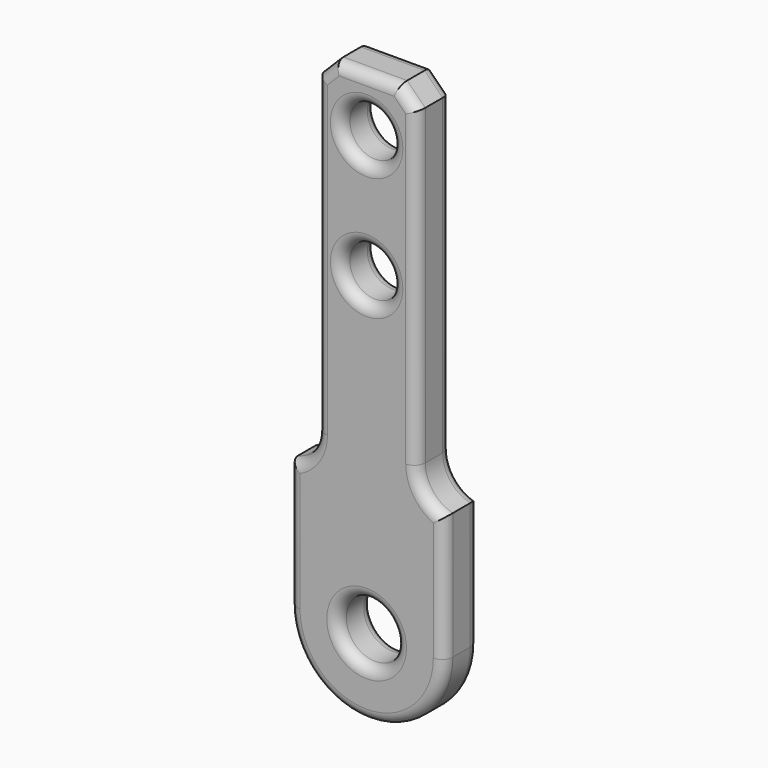
from build123d import *

# Parameters (mm, degrees)
F0_R        = 3.5
F1_DEPTH    = 3
F2_T1_DEPTH = 6
F3_SIZE     = 2.5
F4_R        = 1.5


# Not quite as in the source:
# - a fillet or chamfer that OpenCascade refuses, or shapes differently, is made with other operations: its cross-section is extruded or revolved along the edge and cut away or added


with BuildPart() as f1:
    # F0 (on Front) → F1 (new body, symmetric)
    with BuildSketch(Plane.XZ):
        with BuildLine():
            ThreePointArc((-10.7, 0), (-7.5660425587, -7.5660425587), (0, -10.7))
            ThreePointArc((0, -10.7), (7.5660425587, -7.5660425587), (10.7, 0))
            Line((10.7, 0), (10.7, 17.5))
            Line((10.7, 17.5), (6.9, 17.5))
            Line((6.9, 17.5), (6.9, 68))
            Line((6.9, 68), (-6.9, 68))
            Line((-6.9, 68), (-6.9, 17.5))
            Line((-6.9, 17.5), (-10.7, 17.5))
            Line((-10.7, 17.5), (-10.7, 0))
        make_face()
        with BuildLine():
            ThreePointArc((0, -4), (-2.8284271247, 2.8284271247), (4, 0))
            ThreePointArc((4, 0), (2.8284271247, -2.8284271247), (0, -4))
        make_face(mode=Mode.SUBTRACT)
        with Locations((0, 43.5)):
            Circle(F0_R, mode=Mode.SUBTRACT)
        with Locations((0, 60.5)):
            Circle(F0_R, mode=Mode.SUBTRACT)
    extrude(amount=F1_DEPTH, both=True)

    # F2: fillet of radius 5 on 2 edges, made by hand

    # F2_s2 → F2_t1 (join)
    with BuildSketch(Plane.XZ.offset(-3)):
        with BuildLine():
            ThreePointArc((-10.7, 17.5), (-7.962996063, 19.2716574383), (-6.9, 22.3538644398))
            Line((-6.9, 22.3538644398), (-6.9, 17.5))
            Line((-6.9, 17.5), (-10.7, 17.5))
        make_face()
        with BuildLine():
            ThreePointArc((6.9, 22.3538644398), (7.962996063, 19.2716574383), (10.7, 17.5))
            Line((10.7, 17.5), (6.9, 17.5))
            Line((6.9, 17.5), (6.9, 22.3538644398))
        make_face()
    extrude(amount=F2_T1_DEPTH)

    # F3
    f3_edges = [f1.edges().sort_by_distance(p)[0] for p in [
        (-6.9, 0, 68),
        (6.9, 0, 68),
    ]]
    chamfer(f3_edges, length=F3_SIZE)

    # F4
    f4_edges = [f1.edges().sort_by_distance(p)[0] for p in [
        (6.9, -3, 43.926932),
        (5.65, -3, 66.75),
        (7.962996, -3, 19.271657),
        (0, -3, 68),
        (10.7, -3, 8.75),
        (-5.65, -3, 66.75),
        (0, -3, -10.7),
        (-6.9, -3, 43.926932),
        (-10.7, -3, 8.75),
        (-7.962996, -3, 19.271657),
        (2.828427, -3, -2.828427),
        (-2.828427, -3, 2.828427),
        (-3.5, -3, 43.5),
        (-3.5, -3, 60.5),
        (6.9, 3, 43.926932),
        (5.65, 3, 66.75),
        (7.962996, 3, 19.271657),
        (0, 3, 68),
        (10.7, 3, 8.75),
        (-5.65, 3, 66.75),
        (0, 3, -10.7),
        (-6.9, 3, 43.926932),
        (-10.7, 3, 8.75),
        (-7.962996, 3, 19.271657),
        (2.828427, 3, -2.828427),
        (-2.828427, 3, 2.828427),
        (-3.5, 3, 43.5),
        (-3.5, 3, 60.5),
    ]]
    fillet(f4_edges, radius=F4_R)


solid = f1.part
